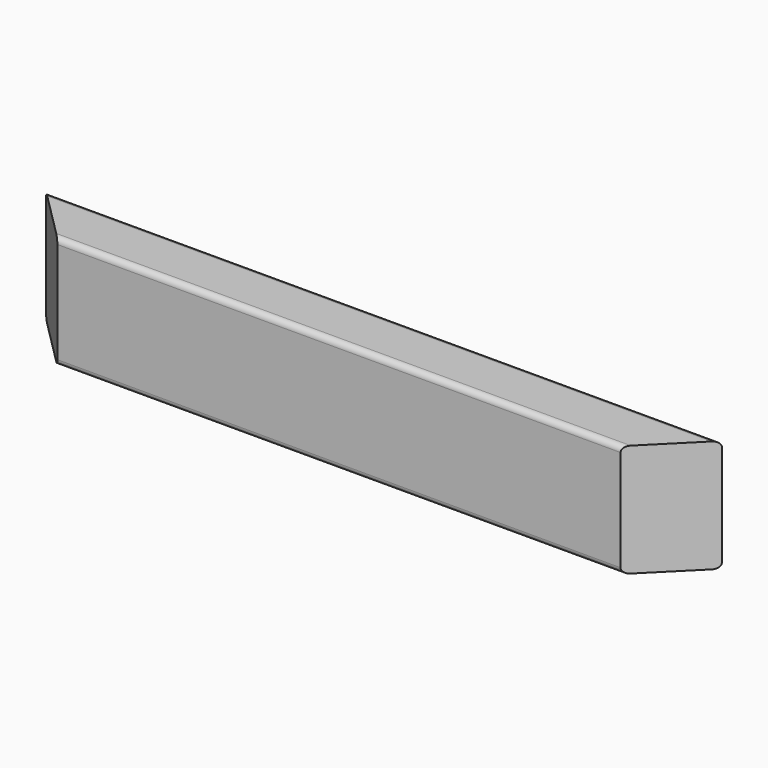
from build123d import *

# Parameters (mm, degrees)
F0_W     = 600
F0_H     = 100
F3_DEPTH = 50
F1_SIZE  = 49.99999
F4_SIZE  = 49.99999
F2_R     = 5


# Not quite as in the source:
# - a fillet or chamfer is up to 0.001 mm smaller than in the source, because OpenCascade refuses the exact size


with BuildPart() as f3:
    # F0 (on Front) → F3 (new body)
    with BuildSketch(Plane.XZ):
        with Locations((-350.3373948519, 50)):
            Rectangle(F0_W, F0_H)
    extrude(amount=F3_DEPTH)

    # F1 (size 50 in the source; OpenCascade refuses exactly that, so slightly less here)
    f1_edges = [f3.edges().sort_by_distance(p)[0] for p in [
        (-50.337395, -50, 50),
    ]]
    chamfer(f1_edges, length=F1_SIZE)

    # F4 (size 50 in the source; OpenCascade refuses exactly that, so slightly less here)
    f4_edges = [f3.edges().sort_by_distance(p)[0] for p in [
        (-650.337395, -50, 50),
    ]]
    chamfer(f4_edges, length=F4_SIZE)

    # F2
    f2_edges = [f3.edges().sort_by_distance(p)[0] for p in [
        (-350.337395, -50, 0),
        (-350.337395, -50, 100),
        (-350.337395, 0, 100),
        (-350.337395, 0, 0),
    ]]
    fillet(f2_edges, radius=F2_R)


solid = f3.part
